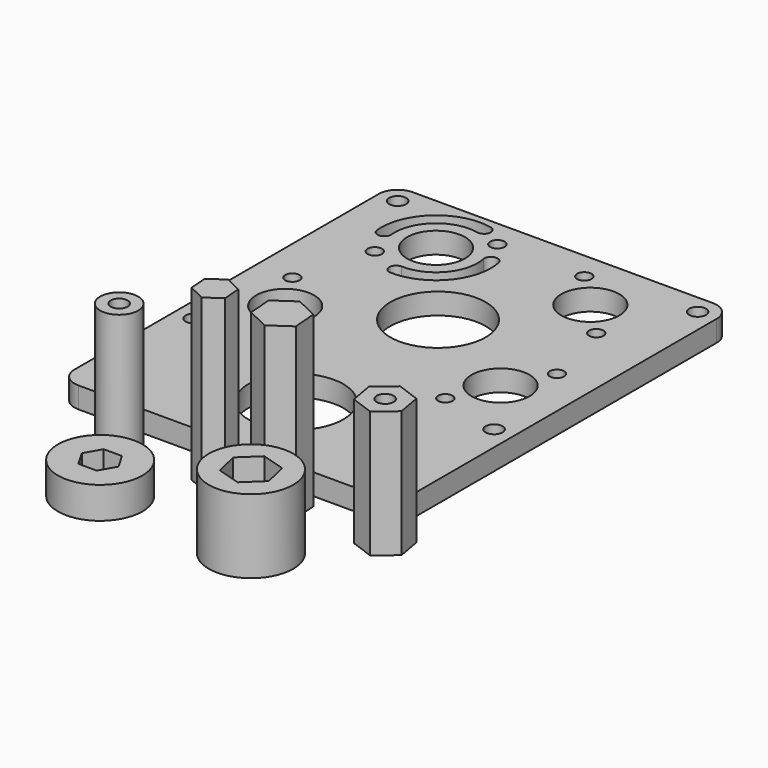
from build123d import *

# Parameters (mm, degrees)
F0_R      = 14.3256
F0_R_2    = 2.54
F0_R_3    = 8.7122
F0_R_4    = 2.159
F1_DEPTH  = 6.35
F2_R      = 5.715
F2_R_2    = 2.54
F3_DEPTH  = 38.1
F5_DEPTH  = 50.8
F6_R      = 12.7
F7_DEPTH  = 9.525
F8_R      = 12.7
F9_DEPTH  = 22.225
F10_R     = 5.715
F11_R     = 2.5527
F12_DEPTH = 38.1


# Not quite as in the source:
# - a length typed as a fraction of an inch, garbled in the dataset ("3 / 203.2 mm" for 3/8 in), is restored


with BuildPart() as f1:
    # F0 (on Top) → F1 (new body)
    with BuildSketch(Plane.XY):
        Polygon((-82.716070006, 115.5439608428), (-82.716070006, 51.6727912001), (-82.716070006, -10.1860391572), (18.883929994, -10.1860391572), (18.883929994, 51.6727912001), (18.883929994, 115.5439608428), align=None)
        with Locations((-31.916070006, 15.2139608428)):
            Circle(F0_R, mode=Mode.SUBTRACT)
        with Locations((-77.001070006, 33.327232354)):
            Circle(F0_R_2, mode=Mode.SUBTRACT)
        with Locations((-64.2949825134, 51.6727912001)):
            Circle(F0_R_3, mode=Mode.SUBTRACT)
        with Locations((-56.6246563405, 39.3636601194)):
            Circle(F0_R_4, mode=Mode.SUBTRACT)
        with Locations((13.168929994, 33.327232354)):
            Circle(F0_R_2, mode=Mode.SUBTRACT)
        with Locations((-5.6086154291, 38.5013823857)):
            Circle(F0_R_4, mode=Mode.SUBTRACT)
        with Locations((0.4628425014, 51.6727912001)):
            Circle(F0_R_3, mode=Mode.SUBTRACT)
        with Locations((-71.9653086863, 63.9819222808)):
            Circle(F0_R_4, mode=Mode.SUBTRACT)
        with Locations((-31.916070006, 68.6301608428)):
            Circle(F0_R, mode=Mode.SUBTRACT)
        with Locations((-65.2144100543, 86.4875327271)):
            Circle(F0_R_4, mode=Mode.SUBTRACT)
        with Locations((-77.001070006, 109.8289608428)):
            Circle(F0_R_2, mode=Mode.SUBTRACT)
        with BuildLine():
            ThreePointArc((-71.5595131301, 95.2740560975), (-66.0899859638, 109.2419811661), (-51.5781883746, 113.0401898065))
            ThreePointArc((-51.5781883746, 113.0401898065), (-50.0260120377, 110.6217612632), (-52.4444405811, 109.0695849263))
            ThreePointArc((-52.4444405811, 109.0695849263), (-63.3895905293, 106.2048837858), (-67.5148406655, 95.6699356926))
            ThreePointArc((-67.5148406655, 95.6699356926), (-69.3392371002, 93.4496596627), (-71.5595131301, 95.2740560975))
        make_face(mode=Mode.SUBTRACT)
        with BuildLine():
            ThreePointArc((-38.8883228105, 100.1269722461), (-42.4749923158, 86.2096266807), (-55.6013943424, 80.3569114506))
            ThreePointArc((-55.6013943424, 80.3569114506), (-57.5711931069, 82.449264391), (-55.4788401666, 84.4190631556))
            ThreePointArc((-55.4788401666, 84.4190631556), (-45.5785891757, 88.8333230296), (-42.8734359851, 99.3301228339))
            ThreePointArc((-42.8734359851, 99.3301228339), (-41.279304104, 101.7211041273), (-38.8883228105, 100.1269722461))
        make_face(mode=Mode.SUBTRACT)
        with Locations((-55.1027520396, 96.8847912001)):
            Circle(F0_R_3, mode=Mode.SUBTRACT)
        with Locations((-44.991094025, 107.2820496732)):
            Circle(F0_R_4, mode=Mode.SUBTRACT)
        with Locations((7.0771174789, 64.5801525913)):
            Circle(F0_R_4, mode=Mode.SUBTRACT)
        with Locations((-8.7293879723, 96.8847912001)):
            Circle(F0_R_3, mode=Mode.SUBTRACT)
        with Locations((-18.841045987, 107.2820496732)):
            Circle(F0_R_4, mode=Mode.SUBTRACT)
        with Locations((1.3822700423, 86.4875327271)):
            Circle(F0_R_4, mode=Mode.SUBTRACT)
        with Locations((13.168929994, 109.8289608428)):
            Circle(F0_R_2, mode=Mode.SUBTRACT)
    extrude(amount=F1_DEPTH)

    # F10
    f10_edges = [f1.edges().sort_by_distance(p)[0] for p in [
        (-82.71607, 115.543961, 3.175),
        (18.88393, 115.543961, 3.175),
        (18.88393, -10.186039, 3.175),
        (-82.71607, -10.186039, 3.175),
    ]]
    fillet(f10_edges, radius=F10_R)


with BuildPart() as f3:
    # F2 (on Top) → F3 (new body)
    with BuildSketch(Plane.XY):
        with Locations((-57.3880523443, -19.3313378841)):
            Circle(F2_R)
        with Locations((-57.3880523443, -19.3313378841)):
            Circle(F2_R_2, mode=Mode.SUBTRACT)
    extrude(amount=F3_DEPTH)


with BuildPart() as f5:
    # F4 (on Top) → F5 (new body)
    with BuildSketch(Plane.XY):
        Polygon((-28.9526027861, -23.8606979485), (-24.4209810199, -20.7452077514), (-24.8532637928, -15.262963083), (-29.8171683318, -12.8962086117), (-34.348790098, -16.0116988088), (-33.9165073252, -21.4939434772), align=None)
    extrude(amount=F5_DEPTH)


with BuildPart() as f5b:
    # F4 (on Top) → F5, piece 2 (new body)
    with BuildSketch(Plane.XY):
        Polygon((-8.5623878158, -25.688112838), (-2.5202254609, -21.5341259085), (-3.0966024913, -14.2244663507), (-9.7151418767, -11.0687937222), (-15.7573042316, -15.2227806517), (-15.1809272012, -22.5324402096), align=None)
    extrude(amount=F5_DEPTH)


with BuildPart() as f7:
    # F6 (on Top) → F7 (new body)
    with BuildSketch(Plane.XY):
        with Locations((-45.5095544457, -41.3338653743)):
            Circle(F6_R)
        Polygon((-40.0102931317, -41.3338653743), (-42.7599237887, -46.0963653743), (-48.2591851028, -46.0963653743), (-51.0088157598, -41.3338653743), (-48.2591851028, -36.5713653743), (-42.7599237887, -36.5713653743), align=None, mode=Mode.SUBTRACT)
    extrude(amount=F7_DEPTH)


with BuildPart() as f9:
    # F8 (on Top) → F9 (new body)
    with BuildSketch(Plane.XY):
        with Locations((0.3517384175, -41.9832840562)):
            Circle(F8_R)
        Polygon((5.6769435627, -36.9428948356), (7.3794461001, -44.074852382), (2.0542409549, -49.1152416026), (-4.9734667277, -47.0236732768), (-6.6759692651, -39.8917157304), (-1.3507641199, -34.8513265098), align=None, mode=Mode.SUBTRACT)
    extrude(amount=F9_DEPTH)


with BuildPart() as f12:
    # F11 (on Top) → F12 (new body)
    with BuildSketch(Plane.XY):
        Polygon((22.934672502, -25.4049720947), (28.5450141377, -20.6840187943), (27.2617194673, -13.4648437637), (20.3680831612, -10.9666220335), (14.7577415256, -15.6875753339), (16.0410361959, -22.9067503645), align=None)
        with Locations((21.6513778316, -18.1857970641)):
            Circle(F11_R, mode=Mode.SUBTRACT)
    extrude(amount=F12_DEPTH)


solid = Compound([f1.part, f3.part, f5.part, f5b.part, f7.part, f9.part, f12.part])
